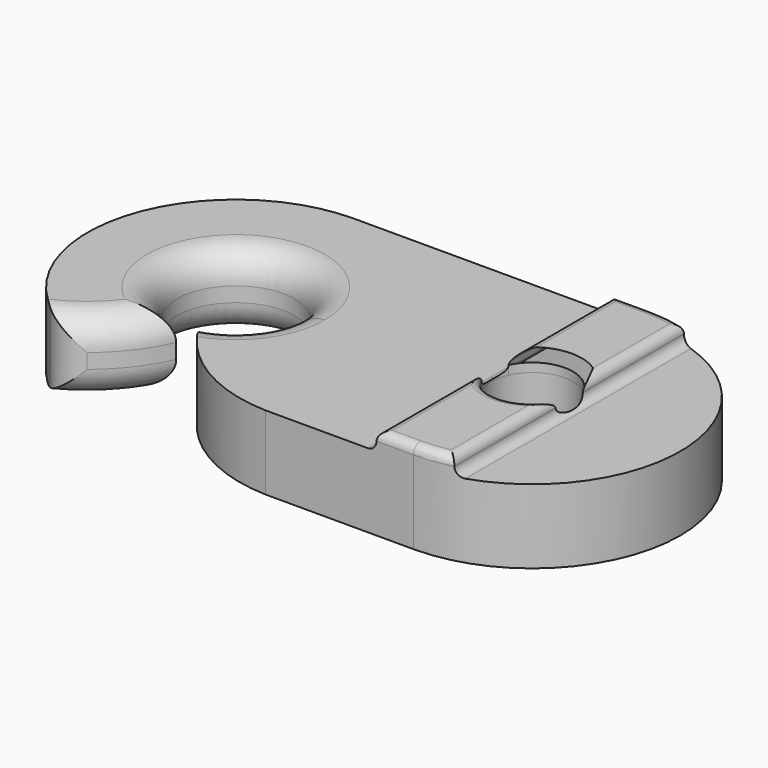
from build123d import *

# Parameters (mm, degrees)
F0_R         = 2.75
F1_DEPTH     = 5
F3_DEPTH     = 1.2
F4_T4_DEPTH  = 10.3543560763
F4_S5_R      = 2.75
F4_T6_DEPTH  = 7
F4_T10_DEPTH = 11.5368144418
F4_S11_R     = 2.75
F4_T12_DEPTH = 7
F4_S13_R     = 10
F4_T14_DEPTH = 7
F4_T18_DEPTH = 10.3543560763
F4_S19_R     = 2.75
F4_T20_DEPTH = 7
F4_T24_DEPTH = 11.5368144418
F4_S25_R     = 10
F4_T26_DEPTH = 7
F4_S27_R     = 2.75
F4_T28_DEPTH = 7
F4_T29_DEPTH = 11.5368144418
F4_T31_DEPTH = 4
F4_T33_DEPTH = 11.8543560763
F4_T35_DEPTH = 11.8543560763
F4_T37_DEPTH = 11.5368144418
F4_T40_ANGLE = 23.0719684246
F4_T42_ANGLE = 193.3175499964
F4_T44_ANGLE = 193.3175499964
F4_T46_ANGLE = 23.0719684246
F5_R         = 2


# Not quite as in the source:
# - a fillet or chamfer that OpenCascade refuses, or shapes differently, is made with other operations: its cross-section is extruded or revolved along the edge and cut away or added


with BuildPart() as f1:
    # F0 (on Top) → F1 (new body)
    with BuildSketch(Plane.XY):
        with BuildLine():
            Line((0, -10), (10, -10))
            ThreePointArc((10, -10), (20, 0), (10, 10))
            Line((10, 10), (0, 10))
            Line((0, 10), (-10, 10))
            ThreePointArc((-10, 10), (-19.6416420475, 2.6530621228), (-15.1159750636, -8.5922522745))
            ThreePointArc((-15.1159750636, -8.5922522745), (-12.6410769035, -6.5743316904), (-10.9, -3.897435054))
            ThreePointArc((-10.9, -3.897435054), (-12.4899799196, 3.1304951685), (-6, 0))
            ThreePointArc((-6, 0), (-6.8695048315, -2.4899799196), (-9.1, -3.897435054))
            ThreePointArc((-9.1, -3.897435054), (-5.4248582308, -8.2532853555), (0, -10))
        make_face()
        with Locations((10, 0)):
            Circle(F0_R, mode=Mode.SUBTRACT)
    extrude(amount=F1_DEPTH)

    # F2 (on face) → F3 (join)
    with BuildSketch(Plane.XY.offset(5)):
        with BuildLine():
            Line((10, 10), (7.5, 10))
            Line((7.5, 10), (7.5, 1.1456439237))
            ThreePointArc((7.5, 1.1456439237), (10, 2.75), (12.5, 1.1456439237))
            Line((12.5, 1.1456439237), (12.5, 9.6824583655))
            ThreePointArc((12.5, 9.6824583655), (11.2600429248, 9.9202969627), (10, 10))
        make_face()
        with BuildLine():
            ThreePointArc((12.5, -1.1456439237), (10, -2.75), (7.5, -1.1456439237))
            Line((7.5, -1.1456439237), (7.5, -10))
            Line((7.5, -10), (10, -10))
            ThreePointArc((10, -10), (11.2600429248, -9.9202969627), (12.5, -9.6824583655))
            Line((12.5, -9.6824583655), (12.5, -1.1456439237))
        make_face()
    extrude(amount=F3_DEPTH)

    # F4: fillet of radius 0.6 on 14 edges, made by hand


with BuildPart() as f4_tool2:
    # F4_s3 → F4_t4 (new body)
    with BuildSketch(Plane.XZ.offset(-10)):
        with BuildLine():
            ThreePointArc((6.9, 5), (7.3242640687, 5.1757359313), (7.5, 5.6))
            Line((7.5, 5.6), (7.5, 5))
            Line((7.5, 5), (6.9, 5))
        make_face()
    extrude(amount=F4_T4_DEPTH)

    # F4_s5 → F4_t6 (cut, symmetric)
    with BuildSketch(Plane.XY.offset(5.3)):
        with Locations((10, 0)):
            Circle(F4_S5_R)
    extrude(amount=F4_T6_DEPTH, both=True, mode=Mode.SUBTRACT)


with BuildPart() as f1_1:
    add(f1.part)

    # F4_t1: union F4_tool2
    add(f4_tool2.part)


with BuildPart() as f4_tool8:
    # F4_s9 → F4_t10 (new body)
    with BuildSketch(Plane.XZ.offset(0.3543560763)):
        with BuildLine():
            ThreePointArc((13.1, 5), (12.6757359313, 5.1757359313), (12.5, 5.6))
            Line((12.5, 5.6), (12.5, 5))
            Line((12.5, 5), (13.1, 5))
        make_face()
    extrude(amount=-F4_T10_DEPTH)

    # F4_s11 → F4_t12 (cut, symmetric)
    with BuildSketch(Plane.XY.offset(5.3)):
        with Locations((10, 0)):
            Circle(F4_S11_R)
    extrude(amount=F4_T12_DEPTH, both=True, mode=Mode.SUBTRACT)

    # F4_s13 → F4_t14 (intersect, symmetric)
    with BuildSketch(Plane.XY.offset(5.3)):
        with Locations((10, 0)):
            Circle(F4_S13_R)
    extrude(amount=F4_T14_DEPTH, both=True, mode=Mode.INTERSECT)


with BuildPart() as f1_2:
    add(f1_1.part)

    # F4_t7: union F4_tool8
    add(f4_tool8.part)


with BuildPart() as f4_tool16:
    # F4_s17 → F4_t18 (new body)
    with BuildSketch(Plane.XZ.offset(-0.3543560763)):
        with BuildLine():
            ThreePointArc((6.9, 5), (7.3242640687, 5.1757359313), (7.5, 5.6))
            Line((7.5, 5.6), (7.5, 5))
            Line((7.5, 5), (6.9, 5))
        make_face()
    extrude(amount=F4_T18_DEPTH)

    # F4_s19 → F4_t20 (cut, symmetric)
    with BuildSketch(Plane.XY.offset(5.3)):
        with Locations((10, 0)):
            Circle(F4_S19_R)
    extrude(amount=F4_T20_DEPTH, both=True, mode=Mode.SUBTRACT)


with BuildPart() as f1_3:
    add(f1_2.part)

    # F4_t15: union F4_tool16
    add(f4_tool16.part)


with BuildPart() as f4_tool22:
    # F4_s23 → F4_t24 (new body)
    with BuildSketch(Plane.XZ.offset(11.1824583655)):
        with BuildLine():
            ThreePointArc((12.5, 5.6), (12.6757359313, 5.1757359313), (13.1, 5))
            Line((13.1, 5), (12.5, 5))
            Line((12.5, 5), (12.5, 5.6))
        make_face()
    extrude(amount=-F4_T24_DEPTH)

    # F4_s25 → F4_t26 (intersect, symmetric)
    with BuildSketch(Plane.XY.offset(5.3)):
        with Locations((10, 0)):
            Circle(F4_S25_R)
    extrude(amount=F4_T26_DEPTH, both=True, mode=Mode.INTERSECT)

    # F4_s27 → F4_t28 (cut, symmetric)
    with BuildSketch(Plane.XY.offset(5.3)):
        with Locations((10, 0)):
            Circle(F4_S27_R)
    extrude(amount=F4_T28_DEPTH, both=True, mode=Mode.SUBTRACT)


with BuildPart() as f1_4:
    add(f1_3.part)

    # F4_t21: union F4_tool22
    add(f4_tool22.part)

    # F4_s30 → F4_t29 (cut)
    with BuildSketch(Plane.XZ.offset(-11.1824583655)):
        with BuildLine():
            ThreePointArc((12.5, 5.6), (12.3242640687, 6.0242640687), (11.9, 6.2))
            Line((11.9, 6.2), (12.5, 6.2))
            Line((12.5, 6.2), (12.5, 5.6))
        make_face()
    extrude(amount=F4_T29_DEPTH, mode=Mode.SUBTRACT)

    # F4_s32 → F4_t31 (cut)
    with BuildSketch(Plane.YZ.offset(6)):
        with BuildLine():
            ThreePointArc((10, 5.6), (9.8242640687, 6.0242640687), (9.4, 6.2))
            Line((9.4, 6.2), (10, 6.2))
            Line((10, 6.2), (10, 5.6))
        make_face()
        with BuildLine():
            ThreePointArc((-10, 5.6), (-9.8242640687, 6.0242640687), (-9.4, 6.2))
            Line((-9.4, 6.2), (-10, 6.2))
            Line((-10, 6.2), (-10, 5.6))
        make_face()
    extrude(amount=F4_T31_DEPTH, mode=Mode.SUBTRACT)

    # F4_s34 → F4_t33 (cut)
    with BuildSketch(Plane.XZ.offset(-11.5)):
        with BuildLine():
            ThreePointArc((8.1, 6.2), (7.6757359313, 6.0242640687), (7.5, 5.6))
            Line((7.5, 5.6), (7.5, 6.2))
            Line((7.5, 6.2), (8.1, 6.2))
        make_face()
    extrude(amount=F4_T33_DEPTH, mode=Mode.SUBTRACT)

    # F4_s36 → F4_t35 (cut)
    with BuildSketch(Plane.XZ.offset(-0.3543560763)):
        with BuildLine():
            ThreePointArc((7.5, 5.6), (7.6757359313, 6.0242640687), (8.1, 6.2))
            Line((8.1, 6.2), (7.5, 6.2))
            Line((7.5, 6.2), (7.5, 5.6))
        make_face()
    extrude(amount=F4_T35_DEPTH, mode=Mode.SUBTRACT)

    # F4_s38 → F4_t37 (cut)
    with BuildSketch(Plane.XZ.offset(-0.3543560763)):
        with BuildLine():
            ThreePointArc((11.9, 6.2), (12.3242640687, 6.0242640687), (12.5, 5.6))
            Line((12.5, 5.6), (12.5, 6.2))
            Line((12.5, 6.2), (11.9, 6.2))
        make_face()
    extrude(amount=F4_T37_DEPTH, mode=Mode.SUBTRACT)

    # F4_s39 → F4_t40 (revolve, cut)
    with BuildSketch(Plane(origin=(8.4642453755, -3.6054131494, 0), x_dir=(0, 0, 1), z_dir=(0.9200133355, -0.3918870532, 0))):
        with BuildLine():
            ThreePointArc((5.6, -13.9188705318), (6.0242640687, -13.7431346005), (6.2, -13.3188705318))
            Line((6.2, -13.3188705318), (6.2, -13.9188705318))
            Line((6.2, -13.9188705318), (5.6, -13.9188705318))
        make_face()
    revolve(axis=Axis((10, 0, 6.2), (0, 0, 1)), revolution_arc=F4_T40_ANGLE, mode=Mode.SUBTRACT)

    # F4_s41 → F4_t42 (revolve, cut)
    with BuildSketch(Plane(origin=(0.1344581916, -1.1517390808, 0), x_dir=(0, 0, 1), z_dir=(0.1159561087, -0.9932543384, 0))):
        with BuildLine():
            ThreePointArc((6.2, -6.5825433845), (6.0242640687, -7.0068074532), (5.6, -7.1825433845))
            Line((5.6, -7.1825433845), (6.2, -7.1825433845))
            Line((6.2, -7.1825433845), (6.2, -6.5825433845))
        make_face()
    revolve(axis=Axis((10, 0, 6.2), (0, 0, -1)), revolution_arc=F4_T42_ANGLE, mode=Mode.SUBTRACT)

    # F4_s43 → F4_t44 (revolve, cut)
    with BuildSketch(Plane(origin=(0.1344581916, -1.1517390808, 0), x_dir=(0, 0, 1), z_dir=(-0.1159561087, 0.9932543384, 0))):
        with BuildLine():
            ThreePointArc((6.2, 13.2825433845), (6.0242640687, 12.8582793158), (5.6, 12.6825433845))
            Line((5.6, 12.6825433845), (6.2, 12.6825433845))
            Line((6.2, 12.6825433845), (6.2, 13.2825433845))
        make_face()
    revolve(axis=Axis((10, 0, 6.2), (0, 0, -1)), revolution_arc=F4_T44_ANGLE, mode=Mode.SUBTRACT)

    # F4_s45 → F4_t46 (revolve, cut)
    with BuildSketch(Plane.YZ.offset(10)):
        with BuildLine():
            ThreePointArc((-9.4, 6.2), (-9.8242640687, 6.0242640687), (-10, 5.6))
            Line((-10, 5.6), (-10, 6.2))
            Line((-10, 6.2), (-9.4, 6.2))
        make_face()
    revolve(axis=Axis((10, 0, 6.2), (0, 0, 1)), revolution_arc=F4_T46_ANGLE, mode=Mode.SUBTRACT)

    # F5
    f5_edges = [f1_4.edges().sort_by_distance(p)[0] for p in [
        (-12.48998, 3.130495, 5),
        (-12.48998, 3.130495, 0),
        (-15.115975, -8.592252, 2.5),
        (0, -10, 2.5),
        (-12.641077, -6.574332, 0),
        (-12.641077, -6.574332, 5),
        (-6.869505, -2.48998, 5),
        (-6.869505, -2.48998, 0),
    ]]
    fillet(f5_edges, radius=F5_R)


solid = f1_4.part
